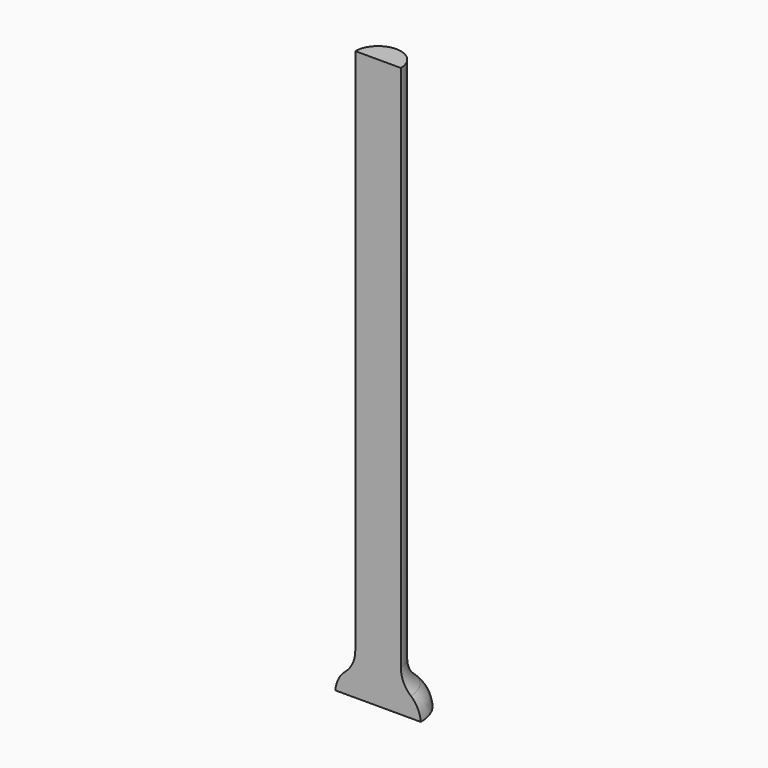
from build123d import *

# Parameters (mm, degrees)
F1_DEPTH    = 5
F2_DEPTH    = 200
F3_T2_ANGLE = 180
F4_T2_ANGLE = 275.6465366004


# Not quite as in the source:
# - a fillet or chamfer that OpenCascade refuses, or shapes differently, is made with other operations: its cross-section is extruded or revolved along the edge and cut away or added


with BuildPart() as f1:
    # F0 (on Top) → F1 (new body)
    with BuildSketch(Plane.XY):
        with BuildLine():
            ThreePointArc((15, 0), (0, 15), (-15, 0))
            Line((-15, 0), (-8, 0))
            ThreePointArc((-8, 0), (0, 8), (8, 0))
            Line((8, 0), (15, 0))
        make_face()
        with BuildLine():
            ThreePointArc((8, 0), (0, 8), (-8, 0))
            Line((-8, 0), (8, 0))
        make_face()
    extrude(amount=F1_DEPTH)

    # F0 (on Top) → F2 (join)
    with BuildSketch(Plane.XY):
        with BuildLine():
            ThreePointArc((8, 0), (0, 8), (-8, 0))
            Line((-8, 0), (8, 0))
        make_face()
    extrude(amount=F2_DEPTH)

    # F3: fillet of radius 10 on 1 edges, made by hand

    # F3_s1 → F3_t2 (revolve)
    with BuildSketch(Plane.XZ):
        with BuildLine():
            ThreePointArc((-8, 14.5393920142), (-9.9377422517, 8.6233122311), (-15, 5))
            Line((-15, 5), (-8, 5))
            Line((-8, 5), (-8, 14.5393920142))
        make_face()
    revolve(axis=Axis((0, 0, 5), (0, 0, -1)), revolution_arc=F3_T2_ANGLE)

    # F4: fillet of radius 10 on 1 edges, made by hand

    # F4_s1 → F4_t2 (revolve, cut)
    with BuildSketch(Plane(origin=(0, 0, 0), x_dir=(0, 0, 1), z_dir=(-0.7410773266, -0.6714196869, 0))):
        with BuildLine():
            ThreePointArc((0, -15), (3.8172075141, -13.9552733931), (6.9301950027, -11.511539409))
            ThreePointArc((6.9301950027, -11.511539409), (5.7894854023, -13.1586020321), (5, -15))
            Line((5, -15), (0, -15))
        make_face()
    revolve(axis=Axis((0, 0, 5), (0, 0, 1)), revolution_arc=F4_T2_ANGLE, mode=Mode.SUBTRACT)


solid = f1.part
